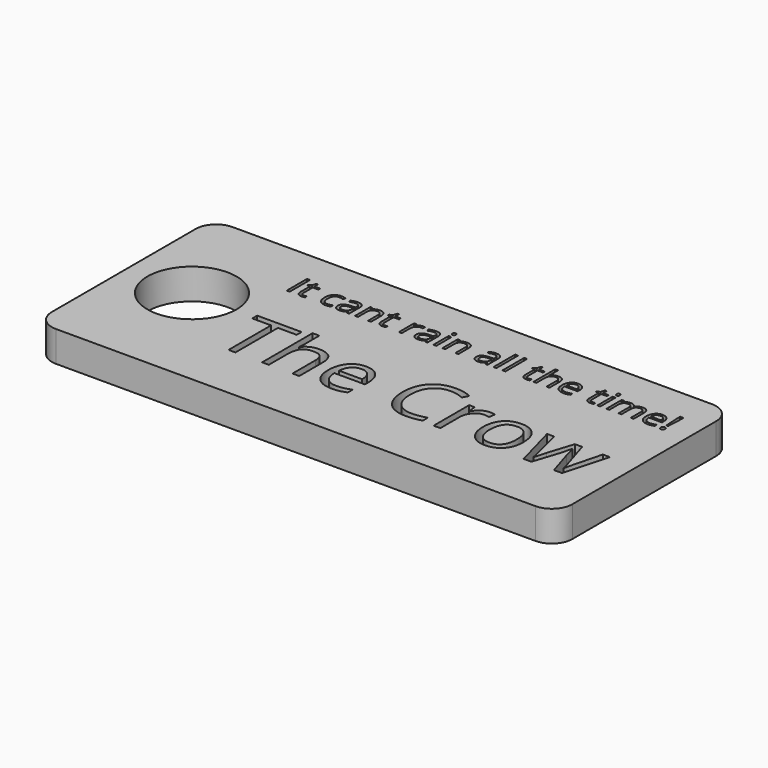
from build123d import *

# Parameters (mm, degrees)
F0_W         = 129.3231025338
F0_H         = 54.8583399504
F1_DEPTH     = 7.62
F2_R         = 11.079876351
F3_DEPTH     = 25.4
F4_R         = 5.08
F5_R         = 5.08
F6_R         = 5.08
F7_TEXT_SIZE = 8.8816833299
F9_DEPTH     = 25.4
F8_TEXT_SIZE = 20.6296422726
F10_DEPTH    = 25.4


# Not quite as in the source:
# - Text() gives the source's letters only with a copy of the font that has no kerning and outlines rounded to 1/6400 em; it was checked with that copy


with BuildPart() as f1:
    # F0 (on Top) → F1 (new body)
    with BuildSketch(Plane.XY):
        with Locations((0.5941353738, 7.9217823222)):
            Rectangle(F0_W, F0_H)
    extrude(amount=F1_DEPTH)

    # F2 (on face) → F3 (cut)
    with BuildSketch(Plane.XY.offset(7.62)):
        with Locations((-47.827757895, 8.812982589)):
            Circle(F2_R)
    extrude(amount=-F3_DEPTH, mode=Mode.SUBTRACT)

    # F4
    f4_edges = [f1.edges().sort_by_distance(p)[0] for p in [
        (65.255687, -19.507388, 3.81),
    ]]
    fillet(f4_edges, radius=F4_R)

    # F5
    f5_edges = [f1.edges().sort_by_distance(p)[0] for p in [
        (65.255687, 35.350952, 3.81),
    ]]
    fillet(f5_edges, radius=F5_R)

    # F6
    f6_edges = [f1.edges().sort_by_distance(p)[0] for p in [
        (-64.067416, 35.350952, 3.81),
        (-64.067416, -19.507388, 3.81),
    ]]
    fillet(f6_edges, radius=F6_R)

    # F7 (on face) → F9 (cut)
    with BuildSketch(Plane.XY.offset(7.62)):
        with Locations((-34.9548656959, 21.0343570464)):
            Text('It cant rain all the time!', F7_TEXT_SIZE, font='Open Sans', text_align=(TextAlign.LEFT, TextAlign.BOTTOM))
    extrude(amount=-F9_DEPTH, mode=Mode.SUBTRACT)

    # F8 (on face) → F10 (cut)
    with BuildSketch(Plane.XY.offset(7.62)):
        with Locations((-32.182238996, -5.4462254047)):
            Text('The Crow', F8_TEXT_SIZE, font='Open Sans', text_align=(TextAlign.LEFT, TextAlign.BOTTOM))
    extrude(amount=-F10_DEPTH, mode=Mode.SUBTRACT)


solid = f1.part
